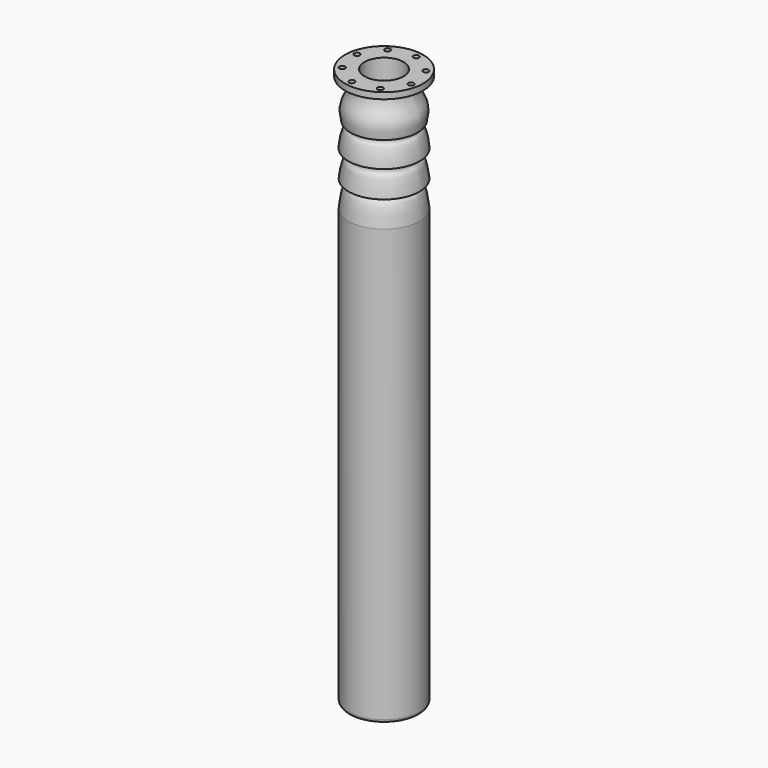
from build123d import *

# Parameters (mm, degrees)
F2_R            = 9
F3_DEPTH        = 20
F3_COPIES_COUNT = 8
F4_R            = 62.5
F5_DEPTH        = 1000
F6_R            = 10


# Not quite as in the source:
# - a pattern or mirror of a feature is missing from the dataset's text; its kind, count and spacing are read off the source's solid
# - a feature names something its author has since deleted; it is built from what else it names


with BuildPart() as f1:
    # F0 (on Front) → F1 (revolve)
    with BuildSketch(Plane.XZ):
        with BuildLine():
            Line((125, 796), (0, 796))
            Line((0, 796), (0, -989))
            Line((0, -989), (113.5784983635, -989))
            Line((113.5784983635, -989), (113.5784983635, 404.0072858334))
            add(Edge.make_bspline(
                [(92.1651435272, 507.9540014267), (92.9137259621, 470.1226269606), (100.84153647, 482.9142285433), (112.1166527424, 426.1022583198), (113.5784983635, 404.0072858334)],
                knots=[0, 0, 0, 0, 0.4424634244, 1, 1, 1, 1], degree=3))
            Line((92.1651435272, 507.9540014267), (113.5784983635, 487.6332684117))
            add(Edge.make_bspline(
                [(92.1651435272, 594.0558493723), (91.8360996428, 546.4974648718), (99.9002877175, 562.9049137477), (112.740117412, 507.2303715025), (113.5784983635, 487.6332684117)],
                knots=[0, 0, 0, 0, 0.4754834111, 1, 1, 1, 1], degree=3))
            Line((92.1651435272, 594.0558493723), (113.8892782108, 573.4401941299))
            add(Edge.make_bspline(
                [(92.1651435272, 666.1855578423), (92.9649518715, 631.6504081509), (100.208934103, 643.7752292593), (113.5784983635, 594.0558493723), (113.8892782108, 573.4401941299)],
                knots=[0, 0, 0, 0, 0.4429655486, 1, 1, 1, 1], degree=3))
            Line((92.1651435272, 666.1855578423), (107.2628746321, 651.8581922678))
            add(Edge.make_bspline(
                [(85, 776), (85.5159944694, 765.5527371234), (86.1594088799, 739.9492330129), (118.4720692878, 693.8768537198), (108.213278463, 662.5958632515), (107.2628746321, 651.8581922678)],
                knots=[0, 0, 0, 0, 0.3013801818, 0.6765769995, 1, 1, 1, 1], degree=3))
            Line((85, 776), (125, 776))
            Line((125, 776), (125, 796))
        make_face()
    revolve(axis=Axis((0, 0, -102), (0, 0, -1)))

    # F2 (on face) → F3 (cut, through all)
    with BuildSketch(Plane.XY.offset(796)):
        with Locations((20.6334079429, 102.9527196176)):
            Circle(F2_R)
    f3 = extrude(amount=-F3_DEPTH, mode=Mode.SUBTRACT)

    # F3_copies: F3 ×8 about axis
    f3_copies_axis = Axis((0, 0, 0), (0, 0, 1))
    for i in range(1, F3_COPIES_COUNT):
        add(f3.rotate(f3_copies_axis, i * 360 / F3_COPIES_COUNT), mode=Mode.SUBTRACT)

    # F4 (on face) → F5 (cut)
    with BuildSketch(Plane.XY.offset(796)):
        Circle(F4_R)
    extrude(amount=-F5_DEPTH, mode=Mode.SUBTRACT)

    # F6
    f6_edges = [f1.edges().sort_by_distance(p)[0] for p in [
        (-113.578498, 0, -989),
    ]]
    fillet(f6_edges, radius=F6_R)


solid = f1.part
